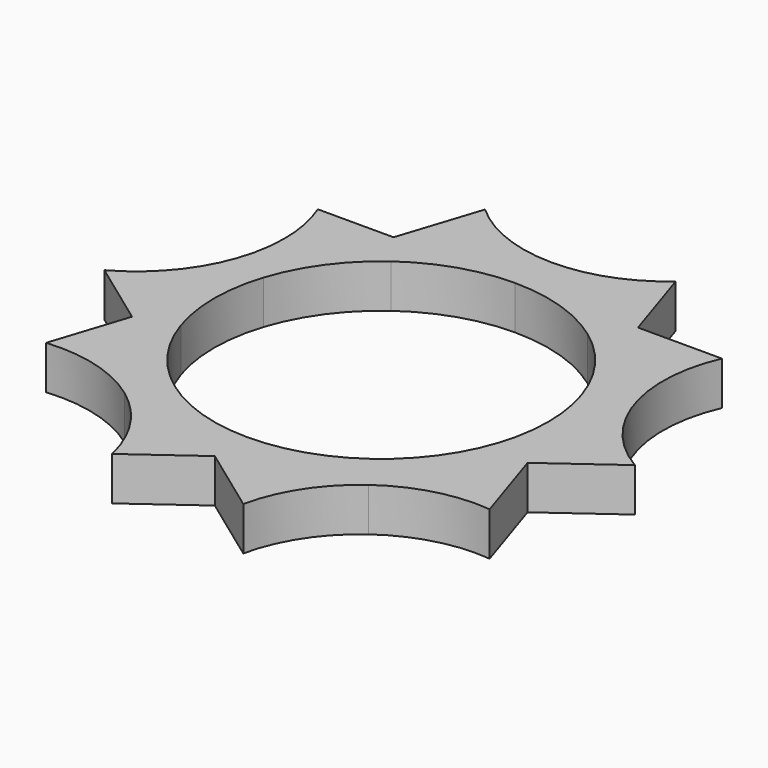
from build123d import *

# Parameters (mm, degrees)
F1_DEPTH = 4


# Not quite as in the source:
# - a feature names something its author has since deleted; it is built from what else it names


with BuildPart() as f1:
    # F0 (on Top) → F1 (new body)
    with BuildSketch(Plane.XY):
        with BuildLine():
            ThreePointArc((-20.4431954222, -12.9176859982), (-15.6048127823, -13.347574962), (-11.2276054917, -15.453473209))
            ThreePointArc((-11.2276054917, -15.453473209), (-7.8721458006, -18.9656863791), (-5.9681546392, -23.4344187216))
            Line((-5.9681546392, -23.4344187216), (0, -19.0983005625))
            Line((0, -19.0983005625), (6.2352903352, -23.6285041655))
            ThreePointArc((6.2352903352, -23.6285041655), (8.0892727444, -19.1867619995), (11.4055803613, -15.6984346018))
            ThreePointArc((11.4055803613, -15.6984346018), (15.747972276, -13.6223910806), (20.5452321785, -13.2317228431))
            Line((20.5452321785, -13.2317228431), (18.1635632001, -5.9016994375))
            Line((18.1635632001, -5.9016994375), (24.3988535354, -1.3714958345))
            ThreePointArc((24.3988535354, -1.3714958345), (18.4546166861, 5.9962684477), (18.9329421283, 15.4508497187))
            Line((18.9329421283, 15.4508497187), (15.537885835, 15.4508497187))
            Line((15.537885835, 15.4508497187), (11.2256994145, 15.4508497187))
            Line((11.2256994145, 15.4508497187), (8.8582927724, 22.7369781668))
            ThreePointArc((8.8582927724, 22.7369781668), (4.7280277023, 20.2947827391), (0, 19.4767594488))
            ThreePointArc((0, 19.4767594488), (-4.7153721091, 20.3911605121), (-8.7986573229, 22.920517208))
            Line((-8.7986573229, 22.920517208), (-11.2256994145, 15.4508497187))
            Line((-11.2256994145, 15.4508497187), (-18.184390629, 15.4508497187))
            ThreePointArc((-18.184390629, 15.4508497187), (-17.4535891597, 12.9689141671), (-17.2070021976, 10.3934006765))
            ThreePointArc((-17.2070021976, 10.3934006765), (-17.4045597984, 8.086010366), (-17.9914818172, 5.8457868068))
            ThreePointArc((-17.9914818172, 5.8457868068), (-20.4374126709, 1.6036270131), (-24.2294812931, -1.4945519715))
            Line((-24.2294812931, -1.4945519715), (-18.1635632001, -5.9016994375))
            Line((-18.1635632001, -5.9016994375), (-20.4431954222, -12.9176859982))
        make_face()
        with BuildLine():
            ThreePointArc((14.5987175251, 4.7434108637), (15.1610160281, 2.4012690384), (15.35, 0))
            ThreePointArc((15.35, 0), (15.1610160281, -2.4012690384), (14.5987175251, -4.7434108637))
            ThreePointArc((14.5987175251, -4.7434108637), (12.4184108637, -9.0225036227), (9.0225036227, -12.4184108637))
            ThreePointArc((9.0225036227, -12.4184108637), (4.7434108637, -14.5987175251), (0, -15.35))
            ThreePointArc((0, -15.35), (-4.7434108637, -14.5987175251), (-9.0225036227, -12.4184108637))
            ThreePointArc((-9.0225036227, -12.4184108637), (-12.4184108637, -9.0225036227), (-14.5987175251, -4.7434108637))
            ThreePointArc((-14.5987175251, -4.7434108637), (-15.35, 0), (-14.5987175251, 4.7434108637))
            ThreePointArc((-14.5987175251, 4.7434108637), (-12.4184108637, 9.0225036227), (-9.0225036227, 12.4184108637))
            ThreePointArc((-9.0225036227, 12.4184108637), (-4.7434108637, 14.5987175251), (0, 15.35))
            ThreePointArc((0, 15.35), (4.7434108637, 14.5987175251), (9.0225036227, 12.4184108637))
            ThreePointArc((9.0225036227, 12.4184108637), (12.4184108637, 9.0225036227), (14.5987175251, 4.7434108637))
        make_face(mode=Mode.SUBTRACT)
    extrude(amount=F1_DEPTH)


solid = f1.part
